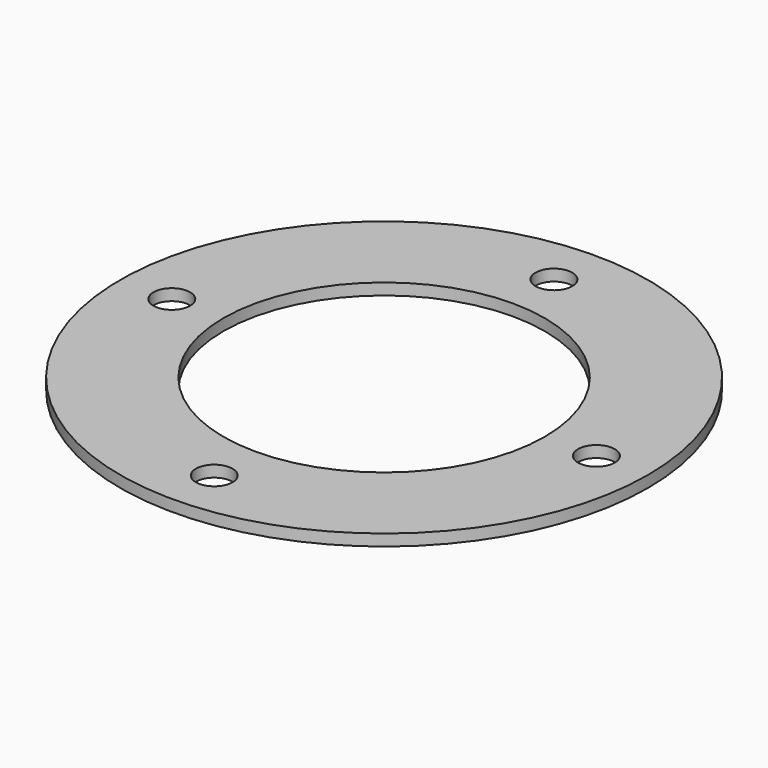
from build123d import *

# Parameters (mm, degrees)
F0_R            = 115
F0_R_2          = 70
F1_DEPTH        = 5
F2_R            = 8
F3_DEPTH        = 25
F3_COPIES_COUNT = 4


# Not quite as in the source:
# - a pattern or mirror of a feature is missing from the dataset's text; its kind, count and spacing are read off the source's solid


with BuildPart() as f1:
    # F0 (on Top) → F1 (new body)
    with BuildSketch(Plane.XY):
        Circle(F0_R)
        Circle(F0_R_2, mode=Mode.SUBTRACT)
    extrude(amount=F1_DEPTH)

    # F2 (on face) → F3 (cut)
    with BuildSketch(Plane.XY.offset(5)):
        with Locations((0, 92.5)):
            Circle(F2_R)
    f3 = extrude(amount=-F3_DEPTH, mode=Mode.SUBTRACT)

    # F3_copies: F3 ×4 about axis
    f3_copies_axis = Axis((0, 0, 0), (0, 0, 1))
    for i in range(1, F3_COPIES_COUNT):
        add(f3.rotate(f3_copies_axis, i * 360 / F3_COPIES_COUNT), mode=Mode.SUBTRACT)


solid = f1.part
